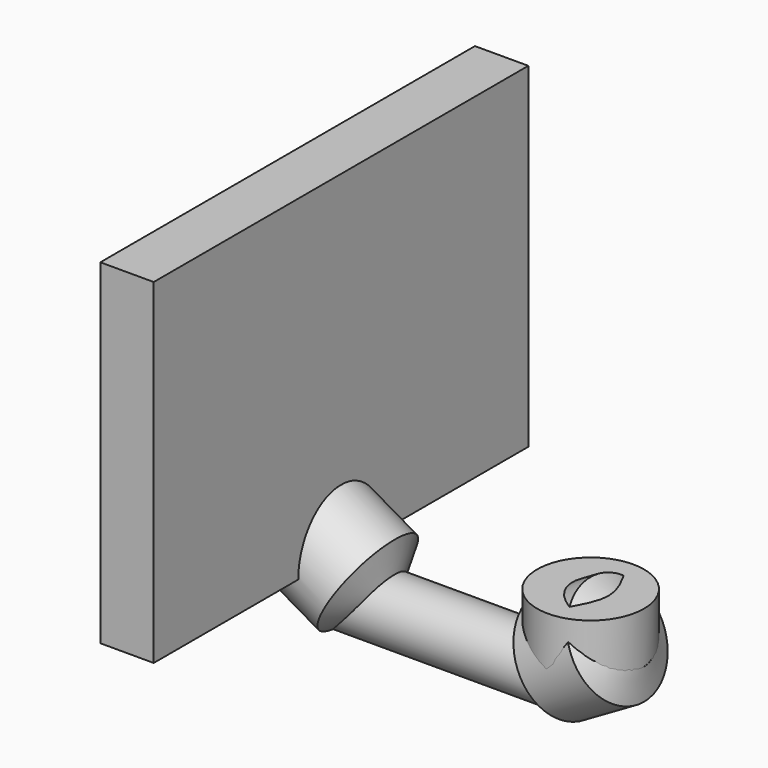
from build123d import *

# Parameters (mm, degrees)
F0_W     = 8.6868
F0_H     = 8.3210518658
F0_H_2   = 54.579148829
F5_DEPTH = 38.1


with BuildPart() as f1:
    # F0 (on Front) → F1 (revolve)
    with BuildSketch(Plane.XZ):
        Polygon((0, 10.0481558442), (0, 5.0240779221), (8.6868, 10.0481558442), align=None)
        Polygon((8.6868, 10.0481558442), (8.6868, 5.0240779221), (17.3736, 5.0240779221), align=None)
        Polygon((8.6868, 10.0481558442), (0, 5.0240779221), (8.6868, 5.0240779221), align=None)
        Polygon((8.6868, 5.0240779221), (0, 5.0240779221), (8.6868, 0), align=None)
        Polygon((17.3736, 5.0240779221), (8.6868, 5.0240779221), (8.6868, 0), align=None)
    revolve(axis=Axis((13.0302, 0, 7.5361168832), (0.8656475241, 0, -0.5006539363)))

    # F0 (on Front) → F5 (join, symmetric)
    with BuildSketch(Plane.XZ):
        with Locations((4.3434, 37.3377302587)):
            Rectangle(F0_W, F0_H_2)
    extrude(amount=F5_DEPTH, both=True)


with BuildPart() as f2:
    # F0 (on Front) → F2 (revolve)
    with BuildSketch(Plane.XZ):
        Polygon((40.6181564641, 5.0240779221), (49.3049564641, 0), (49.3049564641, 5.0240779221), align=None)
        Polygon((49.3049564641, 10.0481558442), (40.6181564641, 5.0240779221), (49.3049564641, 5.0240779221), align=None)
        Polygon((49.3049564641, 5.0240779221), (49.3049564641, 0), (57.9917564641, 5.0240779221), (49.3049564641, 10.0481558442), align=None)
        Polygon((49.3049564641, 10.0481558442), (57.9917564641, 5.0240779221), (57.9917564641, 10.0481558442), align=None)
    revolve(axis=Axis((44.9615564641, 0, 7.5361168832), (-0.8656475241, 0, -0.5006539363)))


with BuildPart() as f3:
    # F0 (on Front) → F3 (revolve)
    with BuildSketch(Plane.XZ):
        Polygon((17.3736, 5.0240779221), (8.6868, 0), (49.3049564641, 0), (40.6181564641, 5.0240779221), align=None)
    revolve(axis=Axis((28.995878232, 0, 5.0240779221), (1, 0, 0)))


with BuildPart() as f4:
    # F0 (on Front) → F4 (revolve)
    with BuildSketch(Plane.XZ):
        with Locations((53.6483564641, 14.2086817771)):
            Rectangle(F0_W, F0_H)
    revolve(axis=Axis((49.3049564641, 0, 11.6966428161), (0, 0, 1)))


solid = Compound([f1.part, f2.part, f3.part, f4.part])
